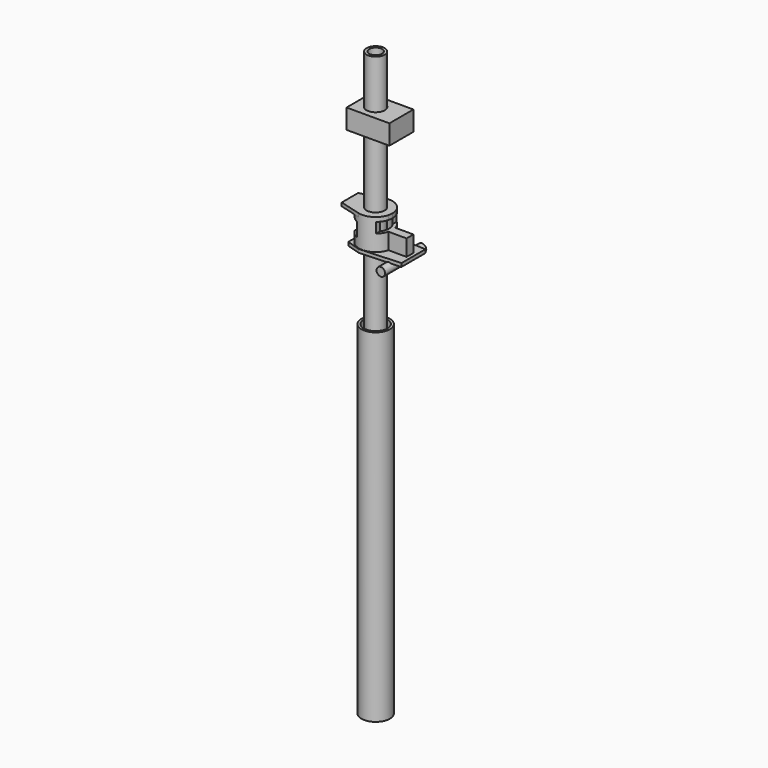
from build123d import *

# Parameters (mm, degrees)
F0_R      = 13.335
F1_DEPTH  = 5.08
F2_DEPTH  = 50.8
F3_DEPTH  = 29.21
F5_DEPTH  = 5.08
F6_R      = 19.685
F7_DEPTH  = 41.275
F9_R      = 13.335
F9_R_2    = 9.525
F10_DEPTH = 457.2
F12_W     = 26.8629424323
F12_H     = 15.24
F13_DEPTH = 50.801
F14_R     = 6.35
F15_DEPTH = 38.1
F16_R     = 7.925577889
F16_R_2   = 6.35
F17_DEPTH = 12.7
F18_W     = 19.05
F18_H     = 19.05
F19_DEPTH = 25.4
F21_R     = 21.082
F21_R_2   = 17.653
F22_DEPTH = 508
F26_SIZE  = 3.175
F28_W     = 63.4833923489
F28_H     = 44.45
F28_R     = 17.4625
F28_R_2   = 13.5255
F29_DEPTH = 3.81
F30_DEPTH = 25.4
F32_DEPTH = 3.81
F33_W     = 19.05
F33_H     = 12.7
F34_DEPTH = 25.4


with BuildPart() as f1:
    # F0 (on Top) → F1 (new body)
    with BuildSketch(Plane.XY):
        Polygon((20.32, 25.4), (0, 19.05), (0, -19.05), (20.32, -25.4), (81.28, -22.225), (81.28, 22.225), align=None)
        with BuildLine():
            ThreePointArc((49.3370575677, -6.35), (0.635, 0), (49.3370575677, 6.35))
            Line((49.3370575677, 6.35), (76.2, 6.35))
            Line((76.2, 6.35), (76.2, -6.35))
            Line((76.2, -6.35), (49.3370575677, -6.35))
        make_face(mode=Mode.SUBTRACT)
        with BuildLine():
            ThreePointArc((49.3370575677, 6.35), (49.9571420941, 3.2018740087), (50.165, 0))
            ThreePointArc((50.165, 0), (49.9571420941, -3.2018740087), (49.3370575677, -6.35))
            Line((49.3370575677, -6.35), (76.2, -6.35))
            Line((76.2, -6.35), (76.2, 6.35))
            Line((76.2, 6.35), (49.3370575677, 6.35))
        make_face()
        with BuildLine():
            ThreePointArc((49.3370575677, -6.35), (49.9571420941, -3.2018740087), (50.165, 0))
            ThreePointArc((50.165, 0), (49.9571420941, 3.2018740087), (49.3370575677, 6.35))
            ThreePointArc((49.3370575677, 6.35), (0.635, 0), (49.3370575677, -6.35))
        make_face()
        with Locations((25.4, 0)):
            Circle(F0_R, mode=Mode.SUBTRACT)
    extrude(amount=F1_DEPTH)

    # F0 (on Top) → F2 (join)
    with BuildSketch(Plane.XY):
        with BuildLine():
            ThreePointArc((49.3370575677, -6.35), (49.9571420941, -3.2018740087), (50.165, 0))
            ThreePointArc((50.165, 0), (49.9571420941, 3.2018740087), (49.3370575677, 6.35))
            ThreePointArc((49.3370575677, 6.35), (0.635, 0), (49.3370575677, -6.35))
        make_face()
        with Locations((25.4, 0)):
            Circle(F0_R, mode=Mode.SUBTRACT)
    extrude(amount=F2_DEPTH)

    # F0 (on Top) → F3 (join)
    with BuildSketch(Plane.XY):
        with BuildLine():
            ThreePointArc((49.3370575677, 6.35), (49.9571420941, 3.2018740087), (50.165, 0))
            ThreePointArc((50.165, 0), (49.9571420941, -3.2018740087), (49.3370575677, -6.35))
            Line((49.3370575677, -6.35), (76.2, -6.35))
            Line((76.2, -6.35), (76.2, 6.35))
            Line((76.2, 6.35), (49.3370575677, 6.35))
        make_face()
    extrude(amount=F3_DEPTH)

    # F4 (on face) → F5 (join)
    with BuildSketch(Plane.XY.offset(50.8)):
        with BuildLine():
            ThreePointArc((18.8567300583, -23.8849501459), (0.6568378159, -1.0397836945), (16.8759001326, 23.2517729743))
            Line((16.8759001326, 23.2517729743), (-12.7, 15.24))
            Line((-12.7, 15.24), (-12.7, -15.24))
            Line((-12.7, -15.24), (18.8567300583, -23.8849501459))
        make_face()
    extrude(amount=-F5_DEPTH)

    # F6 (on face) → F7 (cut)
    with BuildSketch(Plane.XY.offset(5.08)):
        with Locations((25.4, 0)):
            Circle(F6_R)
    extrude(amount=F7_DEPTH, mode=Mode.SUBTRACT)

    # F12 (on offset) → F13 (cut, through all)
    with BuildSketch(Plane.XZ.offset(25.4)):
        Polygon((-14.605, 43.18), (-14.605, 17.78), (15.875, 17.78), (15.875, 38.1), align=None)
        with Locations((54.7064712161, 36.83)):
            Rectangle(F12_W, F12_H)
    extrude(amount=-F13_DEPTH, mode=Mode.SUBTRACT)

    # F14 (on Front) → F15 (join, symmetric)
    with BuildSketch(Plane.XZ):
        with Locations((63.5, -5.588)):
            Circle(F14_R)
    extrude(amount=F15_DEPTH, both=True)

    # F16 (on face) → F17 (cut)
    with BuildSketch(Plane.XZ.offset(38.1)):
        with Locations((63.5, -5.588)):
            Circle(F16_R)
        with Locations((63.5, -5.588)):
            Circle(F16_R_2, mode=Mode.SUBTRACT)
    extrude(amount=-F17_DEPTH, mode=Mode.SUBTRACT)

    # F18 (on Right) → F19 (cut)
    with BuildSketch(Plane.YZ):
        with Locations((0, 14.605)):
            Rectangle(F18_W, F18_H)
    extrude(amount=F19_DEPTH, mode=Mode.SUBTRACT)


with BuildPart() as f10:
    # F9 (on offset) → F10 (new body)
    with BuildSketch(Plane.XY.offset(254)):
        with Locations((25.3833923489, 0)):
            Circle(F9_R)
        with Locations((25.3833923489, 0)):
            Circle(F9_R_2, mode=Mode.SUBTRACT)
    extrude(amount=-F10_DEPTH)


with BuildPart() as f22:
    # F21 (on offset) → F22 (new body)
    with BuildSketch(Plane(origin=(0, 0, -101.6), x_dir=(1, 0, 0), z_dir=(0, 0, -1))):
        with Locations((25.3833923489, 0)):
            Circle(F21_R)
        with Locations((25.3833923489, 0)):
            Circle(F21_R_2, mode=Mode.SUBTRACT)
    extrude(amount=F22_DEPTH)


with BuildPart() as f25:
    # F24 (on plane+point) → F25 (revolve)
    with BuildSketch(Plane.YZ.offset(25.4)):
        Polygon((0, -177.8), (-9.4810361043, -177.8), (-9.4810361043, -203.2), (-17.653, -203.2), (-17.653, -219.075), (0, -219.075), align=None)
    revolve(axis=Axis((25.4, 0, -198.4375), (0, 0, 1)))

    # F26
    f26_edges = [f25.edges().sort_by_distance(p)[0] for p in [
        (25.4, 17.653, -219.075),
        (25.4, 17.653, -203.2),
    ]]
    chamfer(f26_edges, length=F26_SIZE)


with BuildPart() as f29:
    # F28 (on offset) → F29 (new body)
    with BuildSketch(Plane.XY.offset(152.4)):
        with Locations((31.7416961744, 0)):
            Rectangle(F28_W, F28_H)
        with Locations((25.3833923489, 0)):
            Circle(F28_R, mode=Mode.SUBTRACT)
        with Locations((25.3833923489, 0)):
            Circle(F28_R)
        with Locations((25.3833923489, 0)):
            Circle(F28_R_2, mode=Mode.SUBTRACT)
    extrude(amount=F29_DEPTH)

    # F28 (on offset) → F30 (join)
    with BuildSketch(Plane.XY.offset(152.4)):
        with Locations((31.7416961744, 0)):
            Rectangle(F28_W, F28_H)
        with Locations((25.3833923489, 0)):
            Circle(F28_R, mode=Mode.SUBTRACT)
    extrude(amount=F30_DEPTH)

    # F31 (on face) → F32 (join)
    with BuildSketch(Plane.XY.offset(177.8)):
        Polygon((63.4833923489, 22.225), (0, 22.225), (0, 0), (0, -22.225), (63.4833923489, -22.225), align=None)
        with BuildLine():
            ThreePointArc((42.8458923489, 0), (25.3833923489, -17.4625), (7.9208923489, 0))
            ThreePointArc((7.9208923489, 0), (25.3833923489, 17.4625), (42.8458923489, 0))
        make_face(mode=Mode.SUBTRACT)
        with BuildLine():
            ThreePointArc((42.8458923489, 0), (25.3833923489, 17.4625), (7.9208923489, 0))
            ThreePointArc((7.9208923489, 0), (25.3833923489, -17.4625), (42.8458923489, 0))
        make_face()
        with BuildLine():
            ThreePointArc((38.9088923489, 0), (25.3833923489, -13.5255), (11.8578923489, 0))
            ThreePointArc((11.8578923489, 0), (25.3833923489, 13.5255), (38.9088923489, 0))
        make_face(mode=Mode.SUBTRACT)
    extrude(amount=F32_DEPTH)

    # F33 (on face) → F34 (cut)
    with BuildSketch(Plane(origin=(0, 0, 0), x_dir=(0, -1, 0), z_dir=(-1, 0, 0))):
        with Locations((0, 162.56)):
            Rectangle(F33_W, F33_H)
    extrude(amount=-F34_DEPTH, mode=Mode.SUBTRACT)


solid = Compound([f1.part, f10.part, f22.part, f25.part, f29.part])
